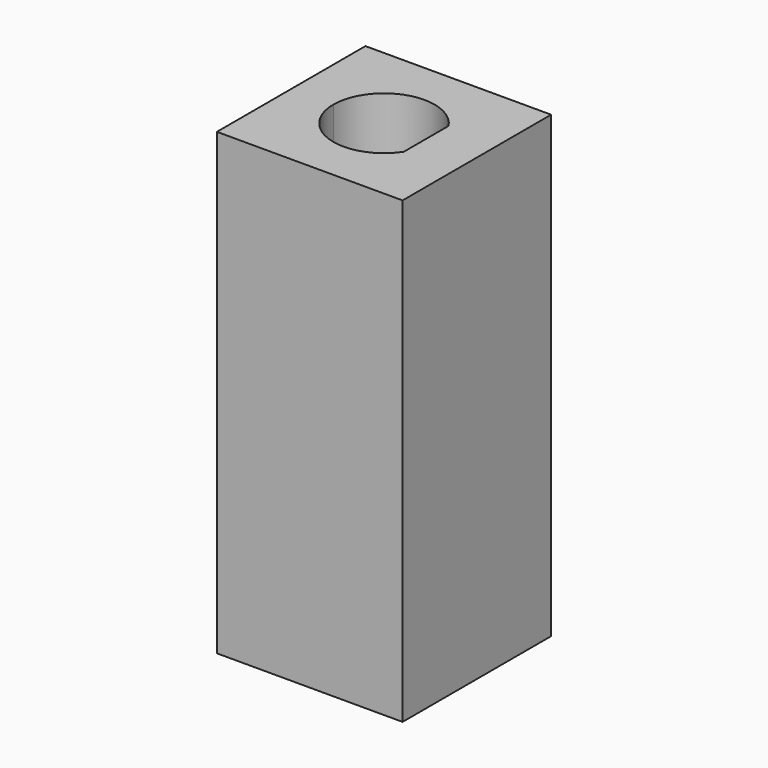
from build123d import *

# Parameters (mm, degrees)
F0_W     = 11
F0_H     = 11
F1_DEPTH = 14.2
F2_W     = 11
F2_H     = 11
F3_DEPTH = 3
F4_W     = 11
F4_H     = 11
F4_W_2   = 3.2
F4_H_2   = 3.2
F5_DEPTH = 10
F6_DEPTH = 25


# Not quite as in the source:
# - a feature names something its author has since deleted; it is built from what else it names


with BuildPart() as f1:
    # F0 (on Top) → F1 (new body)
    with BuildSketch(Plane.XY):
        Rectangle(F0_W, F0_H)
        with BuildLine():
            ThreePointArc((2.5, 1.6583123952), (2.8722813233, 0.8660254038), (3, 0))
            ThreePointArc((3, 0), (2.8722813233, -0.8660254038), (2.5, -1.6583123952))
            ThreePointArc((2.5, -1.6583123952), (-0.8660254038, -2.8722813233), (-3, 0))
            ThreePointArc((-3, 0), (-0.8660254038, 2.8722813233), (2.5, 1.6583123952))
        make_face(mode=Mode.SUBTRACT)
        with BuildLine():
            ThreePointArc((2.5, -1.6583123952), (2.8722813233, -0.8660254038), (3, 0))
            ThreePointArc((3, 0), (2.8722813233, 0.8660254038), (2.5, 1.6583123952))
            Line((2.5, 1.6583123952), (2.5, 0))
            Line((2.5, 0), (2.5, -1.6583123952))
        make_face()
    extrude(amount=F1_DEPTH)

    # F2 (on face) → F3 (join)
    with BuildSketch(Plane(origin=(0, 0, 0), x_dir=(1, 0, 0), z_dir=(0, 0, -1))):
        Rectangle(F2_W, F2_H)
        with BuildLine():
            ThreePointArc((2.5, -1.6583123952), (-3, 0), (2.5, 1.6583123952))
            Line((2.5, 1.6583123952), (2.5, -1.6583123952))
        make_face(mode=Mode.SUBTRACT)
        with BuildLine():
            Line((2.5, -1.6583123952), (2.5, 1.6583123952))
            ThreePointArc((2.5, 1.6583123952), (-3, 0), (2.5, -1.6583123952))
        make_face()
    extrude(amount=F3_DEPTH)

    # F4 (on face) → F5 (join)
    with BuildSketch(Plane(origin=(0, 0, -3), x_dir=(1, 0, 0), z_dir=(0, 0, -1))):
        Rectangle(F4_W, F4_H)
        Rectangle(F4_W_2, F4_H_2, mode=Mode.SUBTRACT)
    extrude(amount=F5_DEPTH)

    # F6 (cut): a face of the model
    f6_faces = [f1.faces().sort_by_distance(p)[0] for p in [
        (0, 0, -3),
    ]]
    extrude(f6_faces, amount=-F6_DEPTH, mode=Mode.SUBTRACT)


solid = f1.part
